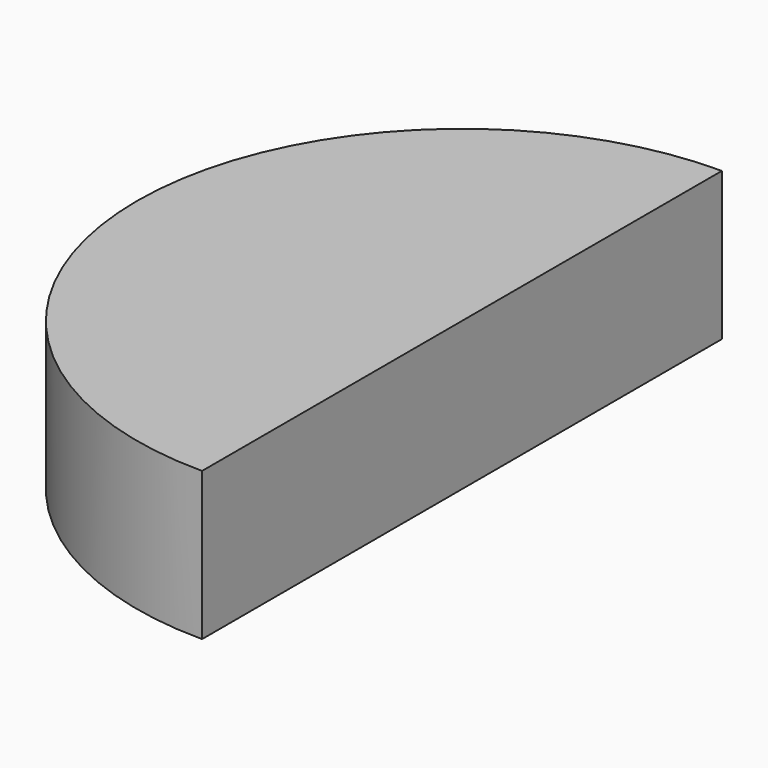
from build123d import *

# Parameters (mm, degrees)
F4_DEPTH = 12.7
F5_R     = 6.1731972722
F6_DEPTH = 12.7
F7_DEPTH = 12.7


# Not quite as in the source:
# - a feature of the source that left no trace in its solid (it failed there, or was rolled back) is left out


with BuildPart() as f4:
    # F3 (on Top) → F4 (new body)
    with BuildSketch(Plane.XY):
        with BuildLine():
            Line((-247.0177412033, 0), (-247.0177412033, 27.8642479823))
            ThreePointArc((-247.0177412033, 27.8642479823), (-274.8819891856, 0), (-247.0177412033, -27.8642479823))
            Line((-247.0177412033, -27.8642479823), (-247.0177412033, 0))
        make_face()
    extrude(amount=F4_DEPTH)

    # F5 (on face) → F6 (join)
    with BuildSketch(Plane.XY.offset(12.7)):
        with Locations((-258.7949037552, 0)):
            Circle(F5_R)
    extrude(amount=-F6_DEPTH)

    # F5 (on face) → F7 (join)
    with BuildSketch(Plane.XY.offset(12.7)):
        with Locations((-258.7949037552, 0)):
            Circle(F5_R)
    extrude(amount=-F7_DEPTH)


solid = f4.part
